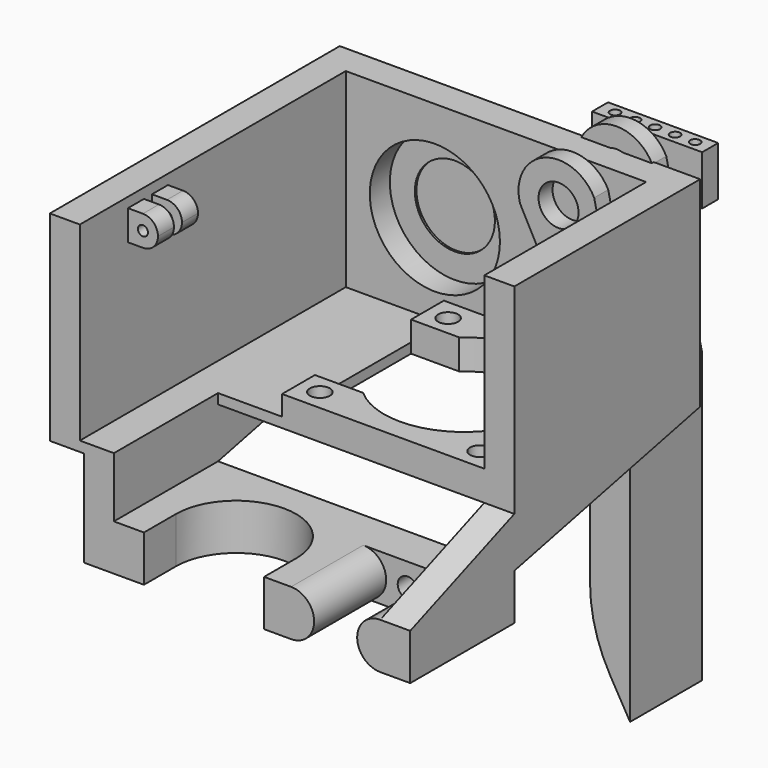
from build123d import *

# Parameters (mm, degrees)
F1_DEPTH  = 20
F0_R      = 1
F2_DEPTH  = 3
F3_R      = 6.5
F3_R_2    = 4
F4_DEPTH  = 2.5
F5_DEPTH  = 2.7
F6_DEPTH  = 1
F9_DEPTH  = 4.6
F11_DEPTH = 3
F13_DEPTH = 3
F14_R     = 1
F14_R_2   = 2
F15_DEPTH = 4.5
F16_DEPTH = 2.75
F17_R     = 1.5
F18_DEPTH = 13
F19_W     = 2
F19_H     = 3
F20_DEPTH = 3
F21_R     = 0.5
F22_DEPTH = 5
F23_W     = 11
F23_H     = 4.9523387714
F24_DEPTH = 2
F25_R     = 0.5
F26_DEPTH = 4
F27_R     = 1
F28_DEPTH = 9
F29_DEPTH = 39.701


# Not quite as in the source:
# - a feature names something its author has since deleted; it is built from what else it names


with BuildPart() as f1:
    # F0 (on Top) → F1 (new body)
    with BuildSketch(Plane.XY):
        Polygon((-20.2, 0), (0, 0), (0, -20.2), (3, -20.2), (3, 3), (-30, 3), (-30, 0), align=None)
        Polygon((-30, -33.2), (-30, 0), (-30, 3), (-33, 3), (-33, -33.2), align=None)
    extrude(amount=F1_DEPTH)

    # F0 (on Top) → F2 (join)
    with BuildSketch(Plane.XY):
        with BuildLine():
            Line((0, -20.2), (0, 0))
            Line((0, 0), (-20.2, 0))
            Line((-20.2, 0), (-20.2, -4.1))
            Line((-20.2, -4.1), (-15.3915026221, -4.1))
            ThreePointArc((-15.3915026221, -4.1), (-6.8084973779, -2.8084973779), (-2.1, -10.1))
            ThreePointArc((-2.1, -10.1), (-6.8084973779, -17.3915026221), (-15.3915026221, -16.1))
            Line((-15.3915026221, -16.1), (-20.2, -16.1))
            Line((-20.2, -16.1), (-20.2, -20.2))
            Line((-20.2, -20.2), (-4, -20.2))
            Line((-4, -20.2), (0, -20.2))
        make_face()
        with Locations((-18.1, -18.1)):
            Circle(F0_R, mode=Mode.SUBTRACT)
        with Locations((-2.1, -18.1)):
            Circle(F0_R, mode=Mode.SUBTRACT)
        with Locations((-18.1, -2.1)):
            Circle(F0_R, mode=Mode.SUBTRACT)
        with Locations((-2.1, -2.1)):
            Circle(F0_R, mode=Mode.SUBTRACT)
    extrude(amount=F2_DEPTH)

    # F3 (on face) → F4 (cut)
    with BuildSketch(Plane.XZ):
        with Locations((-21.1, 10)):
            Circle(F3_R)
        with Locations((-21.1, 10)):
            Circle(F3_R_2, mode=Mode.SUBTRACT)
    extrude(amount=-F4_DEPTH, mode=Mode.SUBTRACT)

    # F3 (on face) → F5 (cut)
    with BuildSketch(Plane.XZ):
        with Locations((-21.1, 10)):
            Circle(F3_R_2)
    extrude(amount=-F5_DEPTH, mode=Mode.SUBTRACT)

    # F0 (on Top) → F6 (join)
    with BuildSketch(Plane.XY):
        Polygon((-20.2, -4.1), (-20.2, 0), (-30, 0), (-30, -33.2), (-26.6, -33.2), (-26.6, -20.2), (-20.2, -20.2), (-20.2, -16.1), align=None)
    extrude(amount=F6_DEPTH)



with BuildPart() as f9:
    # F8 (on offset) → F9 (new body)
    with BuildSketch(Plane.XY.offset(-5)):
        with BuildLine():
            Line((3, -33.2), (3, -20.2))
            Line((3, -20.2), (0, -20.2))
            Line((0, -20.2), (-4, -20.2))
            Line((-4, -20.2), (-20.2, -20.2))
            Line((-20.2, -20.2), (-26.6, -20.2))
            Line((-26.6, -20.2), (-26.6, -33.2))
            Line((-26.6, -33.2), (-23.6, -33.2))
            Line((-23.6, -33.2), (-23.6, -29.2))
            ThreePointArc((-23.6, -29.2), (-17.6, -23.2), (-11.6, -29.2))
            Line((-11.6, -29.2), (-11.6, -33.2))
            Line((-11.6, -33.2), (3, -33.2))
        make_face()
    extrude(amount=-F9_DEPTH)


with BuildPart() as f1_1:
    add(f1.part)

    add(f9.part)  # F11 merges F9
    # F10 (on face) → F11 (join)
    with BuildSketch(Plane.YZ.offset(3)):
        Polygon((3, 0), (-20.2, 0), (-33.2, -5), (-20.2, -5), align=None)
    extrude(amount=-F11_DEPTH)

    # F12 (on face) → F13 (join)
    with BuildSketch(Plane(origin=(-26.6, 0, 0), x_dir=(0, -1, 0), z_dir=(-1, 0, 0))):
        Polygon((33.2, 0), (-3, 0), (20.2, -5), (20.2, -9.6), (33.2, -9.6), (33.2, -5), align=None)
    extrude(amount=F13_DEPTH)

    # F19 (on face) → F20 (join)
    with BuildSketch(Plane.YZ.offset(-30)):
        with Locations((-26.2, 17.5)):
            Rectangle(F19_W, F19_H)
        with Locations((-23.2, 17.5)):
            Rectangle(F19_W, F19_H)
    extrude(amount=F20_DEPTH)

    # F21 (on face) → F22 (cut, through all)
    with BuildSketch(Plane.XZ.offset(27.2)):
        with Locations((-28.5, 17.5)):
            Circle(F21_R)
        with BuildLine():
            ThreePointArc((-28.5, 19), (-27.4393398282, 18.5606601718), (-27, 17.5))
            Line((-27, 17.5), (-27, 19))
            Line((-27, 19), (-28.5, 19))
        make_face()
        with BuildLine():
            ThreePointArc((-27, 17.5), (-27.4393398282, 16.4393398282), (-28.5, 16))
            Line((-28.5, 16), (-27, 16))
            Line((-27, 16), (-27, 17.5))
        make_face()
    extrude(amount=-F22_DEPTH, mode=Mode.SUBTRACT)

    # F27 (on face) → F28 (cut)
    with BuildSketch(Plane.XZ.offset(33.2)):
        with BuildLine():
            Line((0, -5), (-8.9, -5))
            ThreePointArc((-8.9, -5), (-6.6, -7.3), (-8.9, -9.6))
            Line((-8.9, -9.6), (0, -9.6))
            ThreePointArc((0, -9.6), (-2.3, -7.3), (0, -5))
        make_face()
        with Locations((-4.45, -7.3)):
            Circle(F27_R, mode=Mode.SUBTRACT)
        with Locations((-4.45, -7.3)):
            Circle(F27_R)
    extrude(amount=-F28_DEPTH, mode=Mode.SUBTRACT)

    # F27 (on face) → F29 (cut, through all)
    with BuildSketch(Plane.XZ.offset(33.2)):
        with Locations((-4.45, -7.3)):
            Circle(F27_R)
    extrude(amount=-F29_DEPTH, mode=Mode.SUBTRACT)


with BuildPart() as f15:
    # F14 (on Front) → F15 (new body, symmetric)
    with BuildSketch(Plane.XZ):
        with BuildLine():
            Line((2, 3.7956831511), (-0.1009962226, 13.2511583937))
            ThreePointArc((-0.1009962226, 13.2511583937), (-2.7488462539, 11.5272851379), (-5.8849949849, 11.1433321096))
            Line((-5.8849949849, 11.1433321096), (-2, 3.7956831511))
            Line((-2, 3.7956831511), (-2, -14.0525588833))
            ThreePointArc((-2, -14.0525588833), (-1.4888873943, -17.9348445598), (0.0096189432, -21.5525588833))
            Line((0.0096189432, -21.5525588833), (2, -25))
            Line((2, -25), (2, 3.7956831511))
        make_face()
        Circle(F14_R, mode=Mode.SUBTRACT)
        with BuildLine():
            Line((-0.1009962226, 13.2511583937), (-1.5837932006, 19.9244450778))
            ThreePointArc((-1.5837932006, 19.9244450778), (-6.5978749759, 21.8312318779), (-9, 17.0347073736))
            Line((-9, 17.0347073736), (-5.8849949849, 11.1433321096))
            ThreePointArc((-5.8849949849, 11.1433321096), (-2.7488462539, 11.5272851379), (-0.1009962226, 13.2511583937))
        make_face()
        with Locations((-5.14562064, 18.1041744134)):
            Circle(F14_R_2, mode=Mode.SUBTRACT)
    extrude(amount=F15_DEPTH, both=True)

    # F14 (on Front) → F16 (cut, symmetric)
    with BuildSketch(Plane.XZ):
        with BuildLine():
            Line((-0.1009962226, 13.2511583937), (-1.5837932006, 19.9244450778))
            ThreePointArc((-1.5837932006, 19.9244450778), (-6.5978749759, 21.8312318779), (-9, 17.0347073736))
            Line((-9, 17.0347073736), (-5.8849949849, 11.1433321096))
            ThreePointArc((-5.8849949849, 11.1433321096), (-2.7488462539, 11.5272851379), (-0.1009962226, 13.2511583937))
        make_face()
        with Locations((-5.14562064, 18.1041744134)):
            Circle(F14_R_2, mode=Mode.SUBTRACT)
    extrude(amount=F16_DEPTH, both=True, mode=Mode.SUBTRACT)

    # F23 (on face) → F24 (join)
    with BuildSketch(Plane(origin=(0, 4.5, 0), x_dir=(-1, 0, 0), z_dir=(0, 1, 0))):
        with Locations((3.5, 18.9625336896)):
            Rectangle(F23_W, F23_H)
    extrude(amount=F24_DEPTH)

    # F25 (on face) → F26 (cut)
    with BuildSketch(Plane.XY.offset(21.4387030753)):
        with Locations((0.5, 5.5)):
            Circle(F25_R)
        with Locations((-1.5, 5.5)):
            Circle(F25_R)
        with Locations((-3.5, 5.5)):
            Circle(F25_R)
        with Locations((-5.5, 5.5)):
            Circle(F25_R)
        with Locations((-7.5, 5.5)):
            Circle(F25_R)
    extrude(amount=-F26_DEPTH, mode=Mode.SUBTRACT)


with BuildPart() as f18:
    # F17 (on Front) → F18 (new body)
    with BuildSketch(Plane.XZ):
        Circle(F17_R)
    extrude(amount=F18_DEPTH)


solid = Compound([f1_1.part, f15.part, f18.part])
